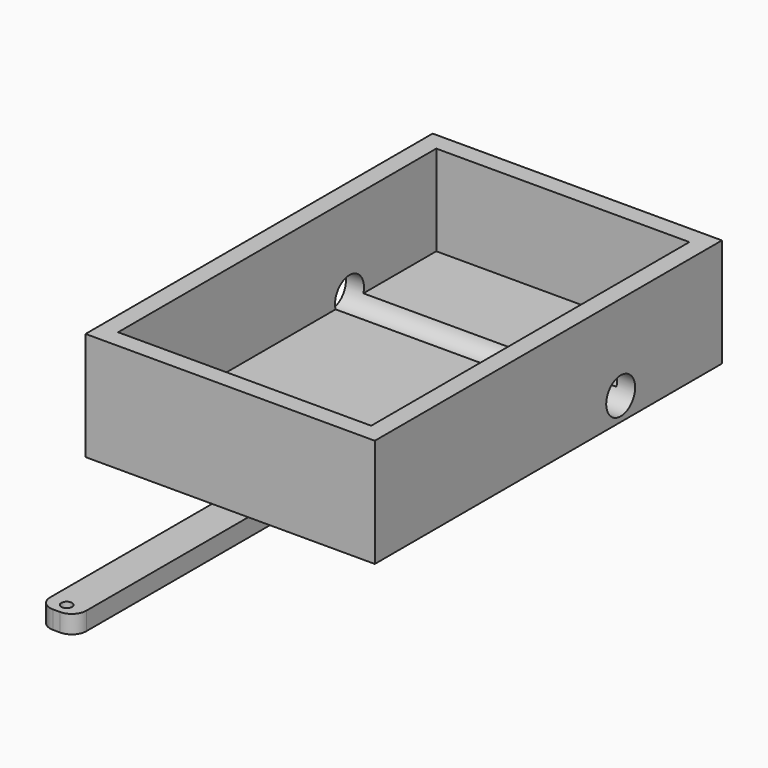
from build123d import *

# Parameters (mm, degrees)
F0_W      = 152.4
F0_H      = 38.1
F1_DEPTH  = 101.6
F2_W      = 88.9
F2_H      = 139.7
F3_DEPTH  = 31.75
F4_R      = 6.35
F5_DEPTH  = 101.6
F6_W      = 12.7
F6_H      = 20.32
F7_DEPTH  = 6.35
F8_W      = 12.7
F8_H      = 6.35
F9_DEPTH  = 76.2
F10_R     = 1.905
F11_DEPTH = 6.35
F12_R     = 5.08


# Not quite as in the source:
# - two fillets or chamfers of one size are made in one step
# - a feature names something its author has since deleted; it is built from what else it names


with BuildPart() as f1:
    # F0 (on Right) → F1 (new body)
    with BuildSketch(Plane.YZ):
        with Locations((3.7253e-06, 2.6738062448)):
            Rectangle(F0_W, F0_H)
    extrude(amount=F1_DEPTH)

    # F2 (on face) → F3 (cut)
    with BuildSketch(Plane.XY.offset(21.7238062448)):
        with Locations((50.8, 3.7253e-06)):
            Rectangle(F2_W, F2_H)
    extrude(amount=-F3_DEPTH, mode=Mode.SUBTRACT)

    # F4 (on face) → F5 (cut)
    with BuildSketch(Plane.YZ.offset(101.6)):
        with Locations((31.7500037253, -8.2481937552)):
            Circle(F4_R)
    extrude(amount=-F5_DEPTH, mode=Mode.SUBTRACT)

    # F6 (on face) → F7 (join)
    with BuildSketch(Plane(origin=(0, 0, -16.3761937552), x_dir=(1, 0, 0), z_dir=(0, 0, -1))):
        with Locations((50.8, 66.0399962747)):
            Rectangle(F6_W, F6_H)
    extrude(amount=F7_DEPTH)

    # F8 (on face) → F9 (join)
    with BuildSketch(Plane.XZ.offset(76.1999962747)):
        with Locations((50.8, -19.5511937552)):
            Rectangle(F8_W, F8_H)
    extrude(amount=F9_DEPTH)

    # F10 (on face) → F11 (cut)
    with BuildSketch(Plane.XY.offset(-16.3761937552)):
        with Locations((50.8, -147.9549962747)):
            Circle(F10_R)
    extrude(amount=-F11_DEPTH, mode=Mode.SUBTRACT)

    # F12
    f12_edges = [f1.edges().sort_by_distance(p)[0] for p in [
        (44.45, -152.399996, -19.551194),
        (57.15, -152.399996, -19.551194),
    ]]
    fillet(f12_edges, radius=F12_R)


solid = f1.part
